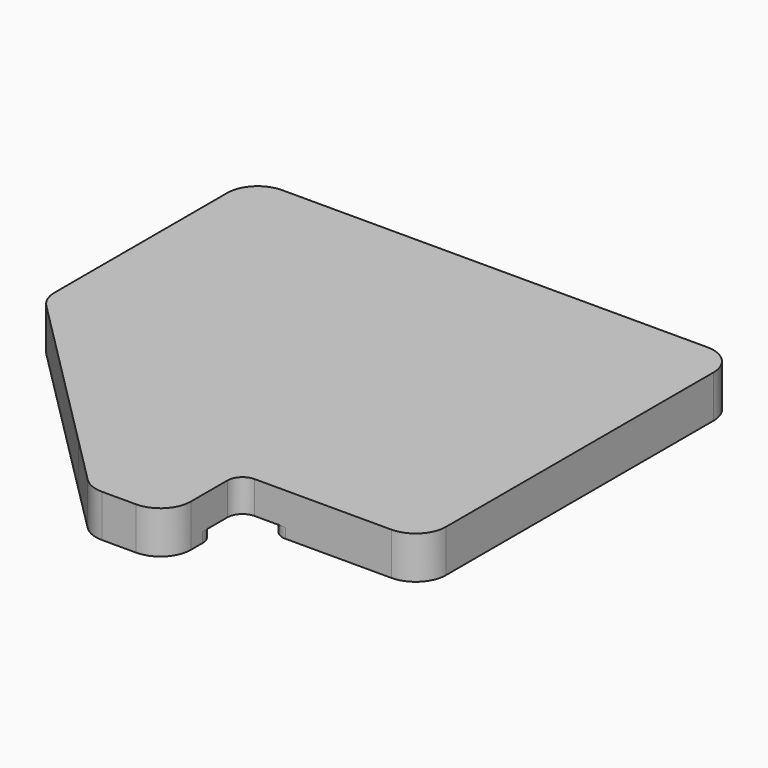
from build123d import *

# Parameters (mm, degrees)
F1_DEPTH = 1.4
F2_START = 0.33
F2_DEPTH = 1.07
F3_R     = 1
F4_F1_R  = 0.5
F4_F2_R  = 0.5


# Not quite as in the source:
# - two fillets or chamfers of one size are made in one step
# - a feature names something its author has since deleted; it is built from what else it names


with BuildPart() as f1:
    # F0 (on Top) → F1 (new body)
    with BuildSketch(Plane.XY):
        Polygon((5.6168799675, 1.8509632612), (7.4634256667, 0), (10, 0), (10, 2.6923049909), (7.9488945061, 0.6460947242), (0.6037752352, 8.0087860049), (7.9664665159, 15.3539052758), (15.3115857869, 7.9912139951), (10.3084311196, 3), (16, 3), (16, 16), (0, 16), (0, 7.4812807055), (2.1561987725, 5.3199235762), align=None)
    extrude(amount=F1_DEPTH)

    # F0 (on Top) → F2 (join)
    with BuildSketch(Plane.XY.offset(F2_START)):
        Polygon((7.9488945061, 0.6460947242), (10, 2.6923049909), (10, 3), (10.3084311196, 3), (15.3115857869, 7.9912139951), (7.9664665159, 15.3539052758), (0.6037752352, 8.0087860049), align=None)
    extrude(amount=F2_DEPTH)

    # F3
    f3_edges = [f1.edges().sort_by_distance(p)[0] for p in [
        (16, 16, 0.7),
        (0, 16, 0.7),
        (10, 0, 0.7),
        (16, 3, 0.7),
        (0, 7.481281, 0.7),
        (7.463426, 0, 0.7),
    ]]
    fillet(f3_edges, radius=F3_R)

    # F4: fillet of radius 0.5 on 7 edges, made by hand

    # F4_f1
    f4_f1_edges = [f1.edges().sort_by_distance(p)[0] for p in [
        (10.3084311196, 3, 0.165),
        (10, 2.6923049909, 0.165),
    ]]
    fillet(f4_f1_edges, radius=F4_F1_R)

    # F4_f2
    f4_f2_edges = [f1.edges().sort_by_distance(p)[0] for p in [
        (7.9664665159, 15.3539052758, 0.165),
        (0.6037752352, 8.0087860049, 0.165),
        (7.9488945061, 0.6460947242, 0.165),
        (15.3115857869, 7.9912139951, 0.165),
        (10, 3, 0.865),
    ]]
    fillet(f4_f2_edges, radius=F4_F2_R)


solid = f1.part
